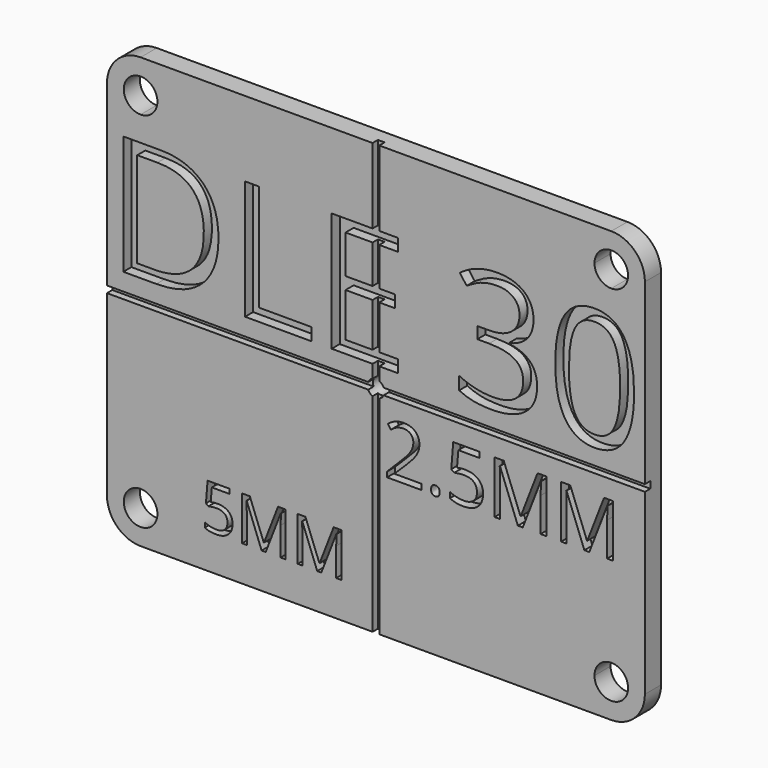
from build123d import *

# Parameters (mm, degrees)
F0_R           = 1.25
F1_DEPTH       = 3
F2_TEXT_SIZE   = 24.8242424242
F3_DEPTH       = 1.5
F4_TEXT_SIZE   = 9.1613778043
F4_TEXT_SIZE_2 = 10.9577270147
F5_DEPTH       = 1.5
F6_W           = 0.5
F6_H           = 6.5202424242
F6_H_2         = 5.7095757576
F6_H_3         = 11.1913285728
F7_DEPTH       = 1


# Not quite as in the source:
# - Text() gives the source's letters only with a copy of the font that has no kerning and outlines rounded to 1/6400 em; it was checked with that copy


with BuildPart() as f1:
    # F0 (on Front) → F1 (new body)
    with BuildSketch(Plane.XZ):
        with BuildLine():
            Line((35, 32), (-35, 32))
            ThreePointArc((-35, 32), (-38.5355339059, 30.5355339059), (-40, 27))
            Line((-40, 27), (-40, -27))
            ThreePointArc((-40, -27), (-38.5355339059, -30.5355339059), (-35, -32))
            Line((-35, -32), (35, -32))
            ThreePointArc((35, -32), (38.5355339059, -30.5355339059), (40, -27))
            Line((40, -27), (40, 27))
            ThreePointArc((40, 27), (38.5355339059, 30.5355339059), (35, 32))
        make_face()
        with BuildLine():
            ThreePointArc((-32.5, -27), (-36.767766953, -28.767766953), (-35, -24.5))
            ThreePointArc((-35, -24.5), (-33.232233047, -25.232233047), (-32.5, -27))
        make_face(mode=Mode.SUBTRACT)
        with BuildLine():
            ThreePointArc((37.5, -27), (35, -29.5), (32.5, -27))
            ThreePointArc((32.5, -27), (33.232233047, -25.232233047), (35, -24.5))
            ThreePointArc((35, -24.5), (36.767766953, -25.232233047), (37.5, -27))
        make_face(mode=Mode.SUBTRACT)
        with BuildLine():
            ThreePointArc((-35, 24.5), (-36.767766953, 28.767766953), (-32.5, 27))
            ThreePointArc((-32.5, 27), (-33.232233047, 25.232233047), (-35, 24.5))
        make_face(mode=Mode.SUBTRACT)
        Circle(F0_R, mode=Mode.SUBTRACT)
        with BuildLine():
            ThreePointArc((35, 24.5), (33.232233047, 25.232233047), (32.5, 27))
            ThreePointArc((32.5, 27), (35, 29.5), (37.5, 27))
            ThreePointArc((37.5, 27), (36.767766953, 25.232233047), (35, 24.5))
        make_face(mode=Mode.SUBTRACT)
    extrude(amount=F1_DEPTH)

    # F2 (on face) → F3 (cut)
    with BuildSketch(Plane.XZ.offset(3)):
        with Locations((-40, 3.086489609)):
            Text('DLE 30', F2_TEXT_SIZE, font='Open Sans', text_align=(TextAlign.LEFT, TextAlign.BOTTOM))
    extrude(amount=-F3_DEPTH, mode=Mode.SUBTRACT)

    # F4 (on face) → F5 (cut)
    with BuildSketch(Plane.XZ.offset(3)):
        with Locations((-26.0373800993, -26.7226658762)):
            Text('5MM', F4_TEXT_SIZE, font='Open Sans', text_align=(TextAlign.LEFT, TextAlign.BOTTOM))
        with Locations((1.1234132107, -11.0728777945)):
            Text('2.5MM', F4_TEXT_SIZE_2, font='Open Sans', text_align=(TextAlign.LEFT, TextAlign.BOTTOM))
    extrude(amount=-F5_DEPTH, mode=Mode.SUBTRACT)

    # F6 (on face) → F7 (cut)
    with BuildSketch(Plane.XZ.offset(3)):
        with BuildLine():
            Line((-1.25, 0), (-40, 0))
            Line((-40, 0), (-40, -0.5))
            Line((-40, -0.5), (-1.1456439237, -0.5))
            ThreePointArc((-1.1456439237, -0.5), (-1.2236328912, -0.2553870546), (-1.25, 0))
        make_face()
        with BuildLine():
            Line((-1.1456439237, 0.5), (-40, 0.5))
            Line((-40, 0.5), (-40, 0))
            Line((-40, 0), (-1.25, 0))
            ThreePointArc((-1.25, 0), (-1.2236328912, 0.2553870546), (-1.1456439237, 0.5))
        make_face()
        with BuildLine():
            ThreePointArc((0, -1.25), (-0.2553870546, -1.2236328912), (-0.5, -1.1456439237))
            Line((-0.5, -1.1456439237), (-0.5, -32))
            Line((-0.5, -32), (0, -32))
            Line((0, -32), (0, -1.25))
        make_face()
        with BuildLine():
            Line((0.5, -32), (0.5, -1.1456439237))
            ThreePointArc((0.5, -1.1456439237), (0.2553870546, -1.2236328912), (0, -1.25))
            Line((0, -1.25), (0, -32))
            Line((0, -32), (0.5, -32))
        make_face()
        with BuildLine():
            Line((40, -0.5), (40, 0))
            Line((40, 0), (1.25, 0))
            ThreePointArc((1.25, 0), (1.2236328912, -0.2553870546), (1.1456439237, -0.5))
            Line((1.1456439237, -0.5), (40, -0.5))
        make_face()
        with BuildLine():
            Line((40, 0), (40, 0.5))
            Line((40, 0.5), (1.1456439237, 0.5))
            ThreePointArc((1.1456439237, 0.5), (1.2236328912, 0.2553870546), (1.25, 0))
            Line((1.25, 0), (40, 0))
        make_face()
        with BuildLine():
            Line((0, 3.086489609), (-0.5, 3.086489609))
            Line((-0.5, 3.086489609), (-0.5, 1.1456439237))
            ThreePointArc((-0.5, 1.1456439237), (-0.2553870546, 1.2236328912), (0, 1.25))
            Line((0, 1.25), (0, 3.086489609))
        make_face()
        with BuildLine():
            Line((0.5, 3.086489609), (0, 3.086489609))
            Line((0, 3.086489609), (0, 1.25))
            ThreePointArc((0, 1.25), (0.2553870546, 1.2236328912), (0.5, 1.1456439237))
            Line((0.5, 1.1456439237), (0.5, 3.086489609))
        make_face()
        with Locations((-0.25, 8.1890350635)):
            Rectangle(F6_W, F6_H)
        with Locations((0.25, 8.1890350635)):
            Rectangle(F6_W, F6_H)
        with Locations((-0.25, 16.1230956696)):
            Rectangle(F6_W, F6_H_2)
        with Locations((0.25, 16.1230956696)):
            Rectangle(F6_W, F6_H_2)
        with Locations((-0.25, 26.4043357136)):
            Rectangle(F6_W, F6_H_3)
        with Locations((0.25, 26.4043357136)):
            Rectangle(F6_W, F6_H_3)
    extrude(amount=-F7_DEPTH, mode=Mode.SUBTRACT)


solid = f1.part
